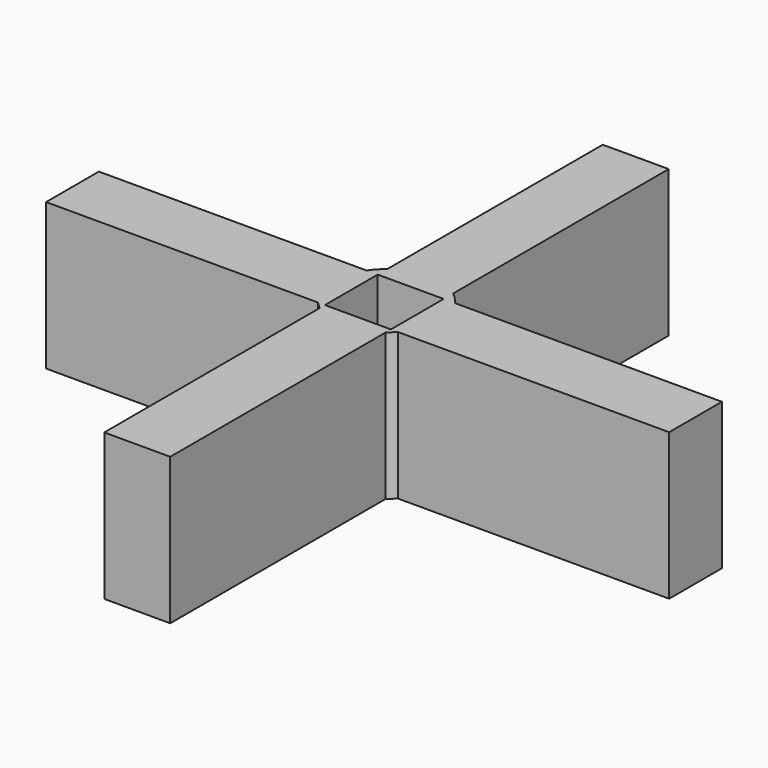
from build123d import *

# Parameters (mm, degrees)
F1_DEPTH = 2


# Not quite as in the source:
# - the program builds the solid bodies; features that only make, move or delete a surface that nothing else refers to are left out


with BuildPart() as f1:
    # F0 (on Top) → F1 (new body)
    with BuildSketch(Plane.XY):
        with BuildLine():
            ThreePointArc((0.5437049493, -0.4874087926), (0.6819795338, -0.2609335518), (0.7301934011, 0))
            ThreePointArc((0.7301934011, 0), (0.697527915, 0.2159565019), (0.6024540634, 0.4125912074))
            Line((0.6024540634, 0.4125912074), (0.45, 0.4125912074))
            Line((0.45, 0.4125912074), (0.45, -0.4874087926))
            Line((0.45, -0.4874087926), (0.5437049493, -0.4874087926))
        make_face()
        with BuildLine():
            ThreePointArc((0.6024540634, 0.4125912074), (0.697527915, 0.2159565019), (0.7301934011, 0))
            ThreePointArc((0.7301934011, 0), (0.6819795338, -0.2609335518), (0.5437049493, -0.4874087926))
            Line((0.5437049493, -0.4874087926), (4.2458724273, -0.4874087926))
            Line((4.2458724273, -0.4874087926), (4.2458724273, 0.4125912074))
            Line((4.2458724273, 0.4125912074), (0.6024540634, 0.4125912074))
        make_face()
        with BuildLine():
            Line((0.45, 0.4125912074), (0.6024540634, 0.4125912074))
            ThreePointArc((0.6024540634, 0.4125912074), (0.5324594789, 0.4996691968), (0.45, 0.5750499134))
            Line((0.45, 0.5750499134), (0.45, 0.4125912074))
        make_face()
        with BuildLine():
            ThreePointArc((0.45, -0.5750499134), (0.4987811374, -0.5332914587), (0.5437049493, -0.4874087926))
            Line((0.5437049493, -0.4874087926), (0.45, -0.4874087926))
            Line((0.45, -0.4874087926), (0.45, -0.5750499134))
        make_face()
        with BuildLine():
            Line((0.45, 0.4125912074), (0.45, 0.5750499134))
            ThreePointArc((0.45, 0.5750499134), (0, 0.7301934011), (-0.45, 0.5750499134))
            Line((-0.45, 0.5750499134), (-0.45, 0.4125912074))
            Line((-0.45, 0.4125912074), (0.45, 0.4125912074))
        make_face()
        with BuildLine():
            ThreePointArc((-0.45, 0.5750499134), (0, 0.7301934011), (0.45, 0.5750499134))
            Line((0.45, 0.5750499134), (0.45, 4.25))
            Line((0.45, 4.25), (-0.45, 4.25))
            Line((-0.45, 4.25), (-0.45, 0.5750499134))
        make_face()
        with BuildLine():
            Line((0.45, -4.25), (0.45, -0.5750499134))
            ThreePointArc((0.45, -0.5750499134), (0, -0.7301934011), (-0.45, -0.5750499134))
            Line((-0.45, -0.5750499134), (-0.45, -4.25))
            Line((-0.45, -4.25), (0.45, -4.25))
        make_face()
        with BuildLine():
            ThreePointArc((-0.45, -0.5750499134), (0, -0.7301934011), (0.45, -0.5750499134))
            Line((0.45, -0.5750499134), (0.45, -0.4874087926))
            Line((0.45, -0.4874087926), (-0.45, -0.4874087926))
            Line((-0.45, -0.4874087926), (-0.45, -0.5750499134))
        make_face()
        with BuildLine():
            Line((-0.45, 0.4125912074), (-0.45, 0.5750499134))
            ThreePointArc((-0.45, 0.5750499134), (-0.5324594789, 0.4996691968), (-0.6024540634, 0.4125912074))
            Line((-0.6024540634, 0.4125912074), (-0.45, 0.4125912074))
        make_face()
        with BuildLine():
            Line((-0.45, -0.4874087926), (-0.45, 0.4125912074))
            Line((-0.45, 0.4125912074), (-0.6024540634, 0.4125912074))
            ThreePointArc((-0.6024540634, 0.4125912074), (-0.7286426563, -0.0475634562), (-0.5437049493, -0.4874087926))
            Line((-0.5437049493, -0.4874087926), (-0.45, -0.4874087926))
        make_face()
        with BuildLine():
            ThreePointArc((-0.5437049493, -0.4874087926), (-0.4987811374, -0.5332914587), (-0.45, -0.5750499134))
            Line((-0.45, -0.5750499134), (-0.45, -0.4874087926))
            Line((-0.45, -0.4874087926), (-0.5437049493, -0.4874087926))
        make_face()
        with BuildLine():
            ThreePointArc((-0.5437049493, -0.4874087926), (-0.7286426563, -0.0475634562), (-0.6024540634, 0.4125912074))
            Line((-0.6024540634, 0.4125912074), (-4.2537945996, 0.4125912074))
            Line((-4.2537945996, 0.4125912074), (-4.2537945996, -0.4874087926))
            Line((-4.2537945996, -0.4874087926), (-0.5437049493, -0.4874087926))
        make_face()
    extrude(amount=F1_DEPTH)


solid = f1.part
